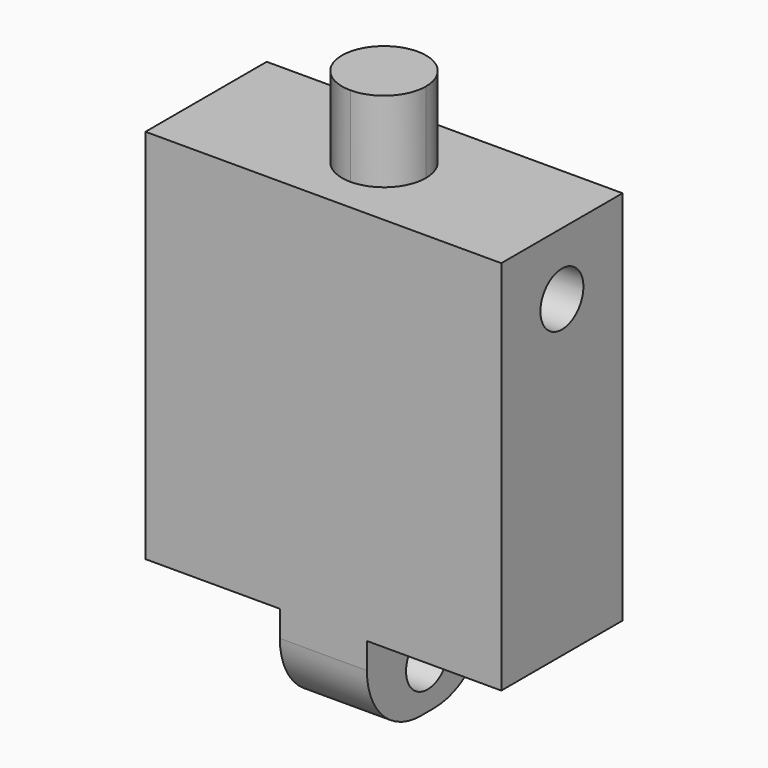
from build123d import *

# Parameters (mm, degrees)
F0_W     = 25.4
F0_H     = 28.6416042886
F0_H_2   = 7.5187312844
F0_H_3   = 21.1228730042
F1_DEPTH = 71.12
F2_DEPTH = 86.36
F3_DEPTH = 17.629891634
F4_R     = 12.7
F6_D     = 10.16
F8_D     = 10.16


with BuildPart() as f1:
    # F0 (on Top) → F1 (new body)
    with BuildSketch(Plane.XY):
        with Locations((-54.5537182136, 5.834735956)):
            Rectangle(F0_W, F0_H)
        with BuildLine():
            Line((-33.6268591068, 20.1555381003), (-41.8537182136, 20.1555381003))
            Line((-41.8537182136, 20.1555381003), (-41.8537182136, -8.4860661883))
            Line((-41.8537182136, -8.4860661883), (-33.6268591068, -8.4860661883))
            Line((-33.6268591068, -8.4860661883), (-33.6268591068, -2.102764044))
            ThreePointArc((-33.6268591068, -2.102764044), (-41.5643591068, 5.834735956), (-33.6268591068, 13.772235956))
            Line((-33.6268591068, 13.772235956), (-33.6268591068, 20.1555381003))
        make_face()
        with BuildLine():
            Line((-25.4, 20.1555381003), (-33.6268591068, 20.1555381003))
            Line((-33.6268591068, 20.1555381003), (-33.6268591068, 13.772235956))
            ThreePointArc((-33.6268591068, 13.772235956), (-28.0141990311, 11.4473960317), (-25.6893591068, 5.834735956))
            ThreePointArc((-25.6893591068, 5.834735956), (-28.0141990311, 0.2220758803), (-33.6268591068, -2.102764044))
            Line((-33.6268591068, -2.102764044), (-33.6268591068, -8.4860661883))
            Line((-33.6268591068, -8.4860661883), (-25.4, -8.4860661883))
            Line((-25.4, -8.4860661883), (-25.4, 12.6368068159))
            Line((-25.4, 12.6368068159), (-25.4, 20.1555381003))
        make_face()
        with Locations((-12.7, 16.3961724581)):
            Rectangle(F0_W, F0_H_2)
        with BuildLine():
            Line((-33.6268591068, -2.102764044), (-33.6268591068, 13.772235956))
            ThreePointArc((-33.6268591068, 13.772235956), (-41.5643591068, 5.834735956), (-33.6268591068, -2.102764044))
        make_face()
        with Locations((-12.7, 2.0753703138)):
            Rectangle(F0_W, F0_H_3)
    extrude(amount=F1_DEPTH)

    # F0 (on Top) → F2 (join)
    with BuildSketch(Plane.XY):
        with BuildLine():
            Line((-33.6268591068, -2.102764044), (-33.6268591068, 13.772235956))
            ThreePointArc((-33.6268591068, 13.772235956), (-41.5643591068, 5.834735956), (-33.6268591068, -2.102764044))
        make_face()
        with BuildLine():
            ThreePointArc((-25.6893591068, 5.834735956), (-28.0141990311, 11.4473960317), (-33.6268591068, 13.772235956))
            Line((-33.6268591068, 13.772235956), (-33.6268591068, -2.102764044))
            ThreePointArc((-33.6268591068, -2.102764044), (-28.0141990311, 0.2220758803), (-25.6893591068, 5.834735956))
        make_face()
    extrude(amount=F2_DEPTH)

    # F0 (on Top) → F3 (join)
    with BuildSketch(Plane.XY):
        with BuildLine():
            ThreePointArc((-25.6893591068, 5.834735956), (-28.0141990311, 11.4473960317), (-33.6268591068, 13.772235956))
            Line((-33.6268591068, 13.772235956), (-33.6268591068, -2.102764044))
            ThreePointArc((-33.6268591068, -2.102764044), (-28.0141990311, 0.2220758803), (-25.6893591068, 5.834735956))
        make_face()
        with BuildLine():
            Line((-25.4, 20.1555381003), (-33.6268591068, 20.1555381003))
            Line((-33.6268591068, 20.1555381003), (-33.6268591068, 13.772235956))
            ThreePointArc((-33.6268591068, 13.772235956), (-28.0141990311, 11.4473960317), (-25.6893591068, 5.834735956))
            ThreePointArc((-25.6893591068, 5.834735956), (-28.0141990311, 0.2220758803), (-33.6268591068, -2.102764044))
            Line((-33.6268591068, -2.102764044), (-33.6268591068, -8.4860661883))
            Line((-33.6268591068, -8.4860661883), (-25.4, -8.4860661883))
            Line((-25.4, -8.4860661883), (-25.4, 12.6368068159))
            Line((-25.4, 12.6368068159), (-25.4, 20.1555381003))
        make_face()
        with BuildLine():
            Line((-33.6268591068, 20.1555381003), (-41.8537182136, 20.1555381003))
            Line((-41.8537182136, 20.1555381003), (-41.8537182136, -8.4860661883))
            Line((-41.8537182136, -8.4860661883), (-33.6268591068, -8.4860661883))
            Line((-33.6268591068, -8.4860661883), (-33.6268591068, -2.102764044))
            ThreePointArc((-33.6268591068, -2.102764044), (-41.5643591068, 5.834735956), (-33.6268591068, 13.772235956))
            Line((-33.6268591068, 13.772235956), (-33.6268591068, 20.1555381003))
        make_face()
        with BuildLine():
            Line((-33.6268591068, -2.102764044), (-33.6268591068, 13.772235956))
            ThreePointArc((-33.6268591068, 13.772235956), (-41.5643591068, 5.834735956), (-33.6268591068, -2.102764044))
        make_face()
    extrude(amount=-F3_DEPTH)

    # F4
    f4_edges = [f1.edges().sort_by_distance(p)[0] for p in [
        (-33.626859, -8.486066, -17.629892),
        (-33.626859, 20.155538, -17.629892),
    ]]
    fillet(f4_edges, radius=F4_R)

    # F6 (through all)
    with Locations(Plane(origin=(-41.8537182136, 0, 0), x_dir=(0, -1, 0), z_dir=(-1, 0, 0))):
        with Locations((-5.834735956, -8.814945817)):
            Hole(F6_D / 2)

    # F8 (through all)
    with Locations(Plane.YZ):
        with Locations((5.834735956, 59.3307428062)):
            Hole(F8_D / 2)


solid = f1.part
